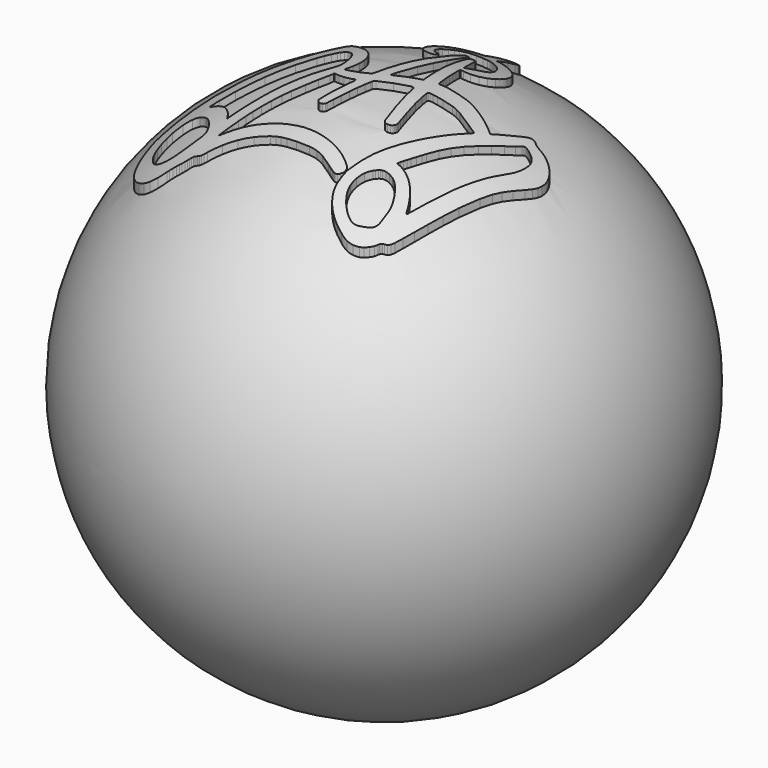
from build123d import *

# Parameters (mm, degrees)
F2_SCALE  = 33.3
F4_DEPTH  = 350
F5_SCALE  = 0.03
F8_SCALE  = 1.4
F9_R      = 2
F10_DEPTH = 25


# Not quite as in the source:
# - ends of sketch curves that miss each other by under 0.0002 mm in the source are joined


with BuildPart() as f1:
    # F0 (on Top) → F1 (revolve)
    with BuildSketch(Plane.XY):
        with BuildLine():
            ThreePointArc((0, 10), (-10, 0), (0, -10))
            Line((0, -10), (0, 10))
        make_face()
    revolve(axis=Axis((0, 0, 0), (0, 1, 0)))


with BuildPart() as f1_1:
    # F2: moved
    add(f1.part.scale(F2_SCALE))

    # F3 (on Top) → F4 (join)
    with BuildSketch(Plane.XY):
        with BuildLine():
            ThreePointArc((16.1837149134, 185.6219143432), (15.1692805921, 185.1870491696), (14.3397748174, 184.4589661515))
            ThreePointArc((14.3397748174, 184.4589661515), (13.6510319308, 183.3784275436), (13.2516433932, 182.1608811178))
            ThreePointArc((13.2516433932, 182.1608811178), (12.7104318622, 179.1680856754), (12.2460595692, 176.1624089195))
            ThreePointArc((12.2460595692, 176.1624089195), (11.7304261477, 172.1284351878), (11.3226162114, 168.0821389815))
            ThreePointArc((11.3226162114, 168.0821389815), (10.8951310079, 162.8117363905), (10.5327134235, 157.536460036))
            Line((10.5327134235, 157.536460036), (9.791164, 145.672526))
            Line((9.791164, 145.672526), (3.780021, 143.498838))
            ThreePointArc((3.780021, 143.498838), (-1.6477610952, 141.1251824988), (-6.7203535297, 138.0651393244))
            ThreePointArc((-6.7203535297, 138.0651393244), (-11.376966369, 134.3574285901), (-15.5191747702, 130.0827038044))
            ThreePointArc((-15.5191747702, 130.0827038044), (-19.0969576158, 125.2903145838), (-22.033620735, 120.0803688722))
            ThreePointArc((-22.033620735, 120.0803688722), (-24.2923210945, 114.5207605988), (-25.8302338375, 108.7202609678))
            ThreePointArc((-25.8302338375, 108.7202609678), (-26.3924557433, 104.1595275807), (-26.2837925551, 99.5655559461))
            ThreePointArc((-26.2837925551, 99.5655559461), (-25.4769738725, 95.4896073492), (-23.8870694152, 91.6507903129))
            ThreePointArc((-23.8870694152, 91.6507903129), (-21.7301657098, 88.5148289409), (-18.934623176, 85.931917761))
            ThreePointArc((-18.934623176, 85.931917761), (-15.6708859709, 84.066137258), (-12.0670000484, 82.9960327237))
            ThreePointArc((-12.0670000484, 82.9960327237), (-9.9514688701, 82.6995503191), (-7.820665005, 82.5477318664))
            ThreePointArc((-7.820665005, 82.5477318664), (-6.2598956775, 82.6218418509), (-4.7338411111, 82.9574763578))
            ThreePointArc((-4.7338411111, 82.9574763578), (-3.6802817431, 83.4443933846), (-2.7901553866, 84.1892094375))
            ThreePointArc((-2.7901553866, 84.1892094375), (-2.1858986044, 85.1009509062), (-1.8924604107, 86.1546550473))
            ThreePointArc((-1.8924604107, 86.1546550473), (-1.8426245804, 86.8806241379), (-1.860013302, 87.6080939788))
            ThreePointArc((-1.860013302, 87.6080939788), (-1.9607246618, 88.1072284011), (-2.1854415077, 88.5641533268))
            ThreePointArc((-2.1854415077, 88.5641533268), (-2.5277112184, 88.9647453673), (-2.9560030801, 89.2716468537))
            ThreePointArc((-2.9560030801, 89.2716468537), (-3.6618204273, 89.6235693148), (-4.392460294, 89.920542189))
            ThreePointArc((-4.392460294, 89.920542189), (-7.1065072138, 91.0410387982), (-9.7123581208, 92.3942217903))
            ThreePointArc((-9.7123581208, 92.3942217903), (-11.4507249242, 93.6626454353), (-12.8778390403, 95.2732859714))
            ThreePointArc((-12.8778390403, 95.2732859714), (-13.8356044552, 97.0406681901), (-14.3428715659, 98.9858249235))
            ThreePointArc((-14.3428715659, 98.9858249235), (-14.521613478, 101.4888433545), (-14.3841001545, 103.9944650183))
            ThreePointArc((-14.3841001545, 103.9944650183), (-13.9482041228, 106.4640083631), (-13.2350706429, 108.8681902312))
            ThreePointArc((-13.2350706429, 108.8681902312), (-12.0847016697, 111.7967649703), (-10.7658611088, 114.6534340541))
            ThreePointArc((-10.7658611088, 114.6534340541), (-9.268237976, 117.4565074493), (-7.6103005428, 120.1678427018))
            ThreePointArc((-7.6103005428, 120.1678427018), (-6.0713916259, 122.2795513115), (-4.3220465667, 124.2205165667))
            ThreePointArc((-4.3220465667, 124.2205165667), (-2.0427283806, 126.2983757659), (0.4185983329, 128.1570475141))
            ThreePointArc((0.4185983329, 128.1570475141), (2.7825294043, 129.5595618954), (5.3085631766, 130.6432455009))
            ThreePointArc((5.3085631766, 130.6432455009), (8.1806159101, 131.4775430213), (11.1293739733, 131.9771082407))
            ThreePointArc((11.1293739733, 131.9771082407), (14.9544272457, 132.2944908395), (18.791164, 132.400393))
            ThreePointArc((18.791164, 132.400393), (21.6806571556, 132.3762113948), (24.5693410001, 132.3036780045))
            ThreePointArc((24.5693410001, 132.3036780045), (26.307751387, 132.1848013044), (28.0336839227, 131.945303557))
            ThreePointArc((28.0336839227, 131.945303557), (29.4825241699, 131.622260103), (30.8949281434, 131.1655213816))
            ThreePointArc((30.8949281434, 131.1655213816), (32.6109340372, 130.4725349399), (34.2911640004, 129.6968200009))
            ThreePointArc((34.2911640004, 129.6968200009), (37.9951081662, 127.5987179258), (41.4287451434, 125.0824961734))
            ThreePointArc((41.4287451434, 125.0824961734), (44.5041115511, 122.2091005808), (47.2099406452, 118.9853187371))
            ThreePointArc((47.2099406452, 118.9853187371), (49.3287125611, 115.6981244902), (51.0020701094, 112.1633380433))
            ThreePointArc((51.0020701094, 112.1633380433), (51.9633429329, 108.8500909146), (52.2845752073, 105.4152019997))
            ThreePointArc((52.2845752073, 105.4152019997), (52.1788202882, 103.3930014318), (51.8679689251, 101.3920390156))
            ThreePointArc((51.8679689251, 101.3920390156), (51.3793933514, 99.7310381661), (50.6292352893, 98.1706238309))
            ThreePointArc((50.6292352893, 98.1706238309), (49.3887670931, 96.267378804), (47.9699187196, 94.4931262474))
            ThreePointArc((47.9699187196, 94.4931262474), (45.1157445833, 91.3136538455), (42.2078228852, 88.1832631085))
            Line((42.2078228852, 88.1832631085), (35.624482, 81.216238))
            Line((35.624482, 81.216238), (31.414756, 95.808316))
            ThreePointArc((31.414756, 95.808316), (30.5747758019, 98.6585264595), (29.7022052286, 101.4989290717))
            ThreePointArc((29.7022052286, 101.4989290717), (28.8907270693, 104.0158337787), (28.0385246844, 106.5192428897))
            ThreePointArc((28.0385246844, 106.5192428897), (27.2982707536, 108.6035005387), (26.5370293603, 110.6801847618))
            ThreePointArc((26.5370293603, 110.6801847618), (26.2437169572, 111.2677894453), (25.8327331947, 111.7800431937))
            ThreePointArc((25.8327331947, 111.7800431937), (25.4802522739, 112.0796118323), (25.0828137789, 112.3163115463))
            ThreePointArc((25.0828137789, 112.3163115463), (24.6227084068, 112.5031852548), (24.141585905, 112.6262294856))
            ThreePointArc((24.141585905, 112.6262294856), (23.6000894231, 112.6925890214), (23.0545419533, 112.6928517741))
            ThreePointArc((23.0545419533, 112.6928517741), (22.4609474828, 112.6292961131), (21.8758000019, 112.5109909925))
            ThreePointArc((21.8758000019, 112.5109909925), (21.2187147252, 112.3098981878), (20.5855640681, 112.0428408591))
            ThreePointArc((20.5855640681, 112.0428408591), (20.1607323375, 111.7679891064), (19.8163702152, 111.3972598449))
            ThreePointArc((19.8163702152, 111.3972598449), (19.5594248386, 110.9371012372), (19.4144355259, 110.4304010782))
            ThreePointArc((19.4144355259, 110.4304010782), (19.3220337791, 109.6802669952), (19.291164, 108.925094))
            ThreePointArc((19.291164, 108.925094), (19.3852916149, 106.0573805668), (19.6672679512, 103.2020119936))
            ThreePointArc((19.6672679512, 103.2020119936), (20.9206581848, 93.8239544773), (22.2043890597, 84.4500020083))
            ThreePointArc((22.2043890597, 84.4500020083), (23.6507956563, 74.229322655), (25.1557427919, 64.0170989687))
            ThreePointArc((25.1557427919, 64.0170989687), (26.6369557977, 54.3850233496), (28.1837279618, 44.7632579937))
            Line((28.1837279618, 44.7632579937), (31.901914, 22.126123))
            Line((31.901914, 22.126123), (26.346539, 19.418249))
            ThreePointArc((26.346539, 19.418249), (24.9715043404, 18.736827914), (23.6055156415, 18.037449689))
            ThreePointArc((23.6055156415, 18.037449689), (21.7119037613, 17.0461943955), (19.8232712195, 16.0454845882))
            ThreePointArc((19.8232712195, 16.0454845882), (17.7770697102, 14.9482118993), (15.7363275839, 13.8408187623))
            ThreePointArc((15.7363275839, 13.8408187623), (13.8353930454, 12.7956894843), (11.9408344366, 11.7390462227))
            ThreePointArc((11.9408344366, 11.7390462227), (10.2357608448, 10.7911533243), (8.5223972402, 9.8583285541))
            ThreePointArc((8.5223972402, 9.8583285541), (7.0602985775, 9.084165839), (5.5872089444, 8.3311271107))
            ThreePointArc((5.5872089444, 8.3311271107), (4.3173161919, 7.6968566116), (3.0447140301, 7.0680399387))
            ThreePointArc((3.0447140301, 7.0680399387), (2.8840367112, 7.0443730497), (2.7395948226, 7.1186288226))
            ThreePointArc((2.7395948226, 7.1186288226), (2.6490578692, 7.2682646369), (2.6382966615, 7.4428270615))
            ThreePointArc((2.6382966615, 7.4428270615), (2.9254660053, 9.0101912635), (3.2173415321, 10.5766859))
            ThreePointArc((3.2173415321, 10.5766859), (3.5670547539, 12.3819405384), (3.9371018372, 14.1831370344))
            ThreePointArc((3.9371018372, 14.1831370344), (4.3905286604, 16.2921707252), (4.8587286662, 18.3979740754))
            ThreePointArc((4.8587286662, 18.3979740754), (7.3036087373, 29.7080586924), (9.5356052963, 41.0620731315))
            ThreePointArc((9.5356052963, 41.0620731315), (11.3297375314, 51.3852863721), (12.8623872203, 61.7505469703))
            ThreePointArc((12.8623872203, 61.7505469703), (14.0102115107, 71.2475265718), (14.8939126099, 80.7727139519))
            ThreePointArc((14.8939126099, 80.7727139519), (15.4313105094, 89.5798061973), (15.6569627413, 98.4003929941))
            ThreePointArc((15.6569627413, 98.4003929941), (15.6890275218, 103.7849560825), (15.7002231557, 109.1696030001))
            ThreePointArc((15.7002231557, 109.1696030001), (15.6481165696, 111.1118828833), (15.4913986894, 113.0485309664))
            ThreePointArc((15.4913986894, 113.0485309664), (15.2950166397, 113.9935034148), (14.919798785, 114.8827448835))
            ThreePointArc((14.919798785, 114.8827448835), (14.4487941297, 115.4056098827), (13.7911639712, 115.6561207748))
            ThreePointArc((13.7911639712, 115.6561207748), (13.3636113076, 115.6929881735), (12.9344749984, 115.694576043))
            ThreePointArc((12.9344749984, 115.694576043), (12.4729567999, 115.6620658314), (12.0145709854, 115.5993090859))
            ThreePointArc((12.0145709854, 115.5993090859), (11.5887291287, 115.5117299525), (11.1697992405, 115.3955012347))
            ThreePointArc((11.1697992405, 115.3955012347), (10.8507606005, 115.2707067502), (10.5516966736, 115.1036135006))
            ThreePointArc((10.5516966736, 115.1036135006), (10.1768291835, 114.7430744846), (9.9606132353, 114.2700369423))
            ThreePointArc((9.9606132353, 114.2700369423), (9.2991267255, 111.5350836806), (8.6559357265, 108.7957700633))
            ThreePointArc((8.6559357265, 108.7957700633), (7.9317638824, 105.5484568402), (7.2587524522, 102.2901561087))
            ThreePointArc((7.2587524522, 102.2901561087), (6.5246468823, 98.4896960964), (5.8286649433, 94.6820700101))
            ThreePointArc((5.8286649433, 94.6820700101), (3.2390112568, 80.4502627726), (0.5295064699, 66.2407861034))
            ThreePointArc((0.5295064699, 66.2407861034), (-2.6948106938, 49.9526915591), (-6.0100623355, 33.6828620693))
            ThreePointArc((-6.0100623355, 33.6828620693), (-9.4598472935, 17.0258658736), (-12.9233232351, 0.371711049))
            ThreePointArc((-12.9233232351, 0.371711049), (-13.3605462648, -0.8244338456), (-14.1215245934, -1.8456284066))
            ThreePointArc((-14.1215245934, -1.8456284066), (-14.298805794, -1.991284186), (-14.5009786768, -2.0997757755))
            ThreePointArc((-14.5009786768, -2.0997757755), (-15.4717200684, -2.5016106982), (-16.4443961129, -2.8987397215))
            ThreePointArc((-16.4443961129, -2.8987397215), (-17.5933724189, -3.357741385), (-18.7470091084, -3.804900716))
            ThreePointArc((-18.7470091084, -3.804900716), (-20.067808676, -4.3038158125), (-21.3920379976, -4.7935550064))
            ThreePointArc((-21.3920379976, -4.7935550064), (-24.693503143, -5.8648357681), (-28.0651240346, -6.6891458318))
            ThreePointArc((-28.0651240346, -6.6891458318), (-31.925581958, -7.3800215193), (-35.8164370636, -7.8716423663))
            ThreePointArc((-35.8164370636, -7.8716423663), (-39.1746262166, -8.1377523396), (-42.5410049916, -8.2632235157))
            ThreePointArc((-42.5410049916, -8.2632235157), (-43.3114521438, -7.86442986), (-43.4025439079, -7.0016860377))
            ThreePointArc((-43.4025439079, -7.0016860377), (-41.8130495855, -2.5451973195), (-40.641365393, 2.0388990813))
            ThreePointArc((-40.641365393, 2.0388990813), (-39.9495299937, 6.5434580932), (-39.7259944757, 11.0953499988))
            ThreePointArc((-39.7259944757, 11.0953499988), (-39.9736025735, 15.4953280542), (-40.6907613549, 19.8435231423))
            ThreePointArc((-40.6907613549, 19.8435231423), (-41.858302321, 23.9893435365), (-43.493257789, 27.974051622))
            ThreePointArc((-43.493257789, 27.974051622), (-45.8358535005, 32.1828815852), (-48.6740508408, 36.0747501317))
            ThreePointArc((-48.6740508408, 36.0747501317), (-52.0247211521, 39.6828979629), (-55.7654615455, 42.8848635969))
            ThreePointArc((-55.7654615455, 42.8848635969), (-59.9662832556, 45.7305331977), (-64.4556810239, 48.0948609477))
            ThreePointArc((-64.4556810239, 48.0948609477), (-69.3196757609, 50.0321037845), (-74.3538649509, 51.4702602117))
            ThreePointArc((-74.3538649509, 51.4702602117), (-77.5971585248, 52.060235073), (-80.8820409982, 52.3369490499))
            ThreePointArc((-80.8820409982, 52.3369490499), (-82.9473411991, 52.0505112999), (-84.7913459515, 51.0772909374))
            ThreePointArc((-84.7913459515, 51.0772909374), (-86.7701676601, 49.231226631), (-88.3813987235, 47.0569168318))
            ThreePointArc((-88.3813987235, 47.0569168318), (-91.9069280027, 41.156453721), (-95.3378537719, 35.2004844365))
            ThreePointArc((-95.3378537719, 35.2004844365), (-99.490595888, 28.010177071), (-103.7735608571, 20.8966689122))
            ThreePointArc((-103.7735608571, 20.8966689122), (-108.7531882179, 12.9064292235), (-113.8324117533, 4.9791278397))
            ThreePointArc((-113.8324117533, 4.9791278397), (-120.3277806536, -4.917768916), (-126.9160680745, -14.7530549496))
            ThreePointArc((-126.9160680745, -14.7530549496), (-135.9712787588, -28.0792936439), (-145.0774889955, -41.3707350031))
            ThreePointArc((-145.0774889955, -41.3707350031), (-153.20486316, -53.2582674065), (-161.2634160329, -65.1925609779))
            ThreePointArc((-161.2634160329, -65.1925609779), (-167.2375766356, -74.2246819748), (-173.0909778416, -83.3355271003))
            ThreePointArc((-173.0909778416, -83.3355271003), (-177.563070075, -90.5376655525), (-181.9087261093, -97.816791936))
            ThreePointArc((-181.9087261093, -97.816791936), (-185.2879018817, -103.8114638517), (-188.4712984623, -109.9123577682))
            ThreePointArc((-188.4712984623, -109.9123577682), (-190.2540089518, -113.5255935339), (-191.9903037715, -117.1613616376))
            ThreePointArc((-191.9903037715, -117.1613616376), (-192.7930450128, -119.0638070124), (-193.4417981706, -121.024115951))
            ThreePointArc((-193.4417981706, -121.024115951), (-193.879582697, -122.8798340455), (-194.1371780105, -124.7690109991))
            ThreePointArc((-194.1371780105, -124.7690109991), (-194.3739822626, -127.8947928847), (-194.5368125893, -131.0253000165))
            ThreePointArc((-194.5368125893, -131.0253000165), (-194.3823750031, -138.2436150808), (-193.3429853893, -145.3883748724))
            ThreePointArc((-193.3429853893, -145.3883748724), (-191.4753146978, -151.7792971079), (-188.633494165, -157.8006040943))
            ThreePointArc((-188.633494165, -157.8006040943), (-184.9737479765, -163.1446659147), (-180.4982857453, -167.8268637135))
            ThreePointArc((-180.4982857453, -167.8268637135), (-175.1554159196, -171.9267200048), (-169.2776890554, -175.2141821185))
            ThreePointArc((-169.2776890554, -175.2141821185), (-165.0035576963, -176.9300756149), (-160.5646198449, -178.1582122865))
            ThreePointArc((-160.5646198449, -178.1582122865), (-156.3827311483, -178.7545456112), (-152.1585579711, -178.741581383))
            ThreePointArc((-152.1585579711, -178.741581383), (-147.9897477257, -178.1200783399), (-143.9546518648, -176.9021923531))
            ThreePointArc((-143.9546518648, -176.9021923531), (-139.7773284426, -175.0248897158), (-135.8390842742, -172.6872565926))
            ThreePointArc((-135.8390842742, -172.6872565926), (-134.6684659752, -171.9217841853), (-133.4780123266, -171.1875394545))
            ThreePointArc((-133.4780123266, -171.1875394545), (-132.02357575, -170.3317183771), (-130.556336222, -169.4980376022))
            ThreePointArc((-130.556336222, -169.4980376022), (-129.066933111, -168.681346713), (-127.565344933, -167.8872821291))
            ThreePointArc((-127.565344933, -167.8872821291), (-126.2831509664, -167.2417808419), (-124.9852508797, -166.628471263))
            ThreePointArc((-124.9852508797, -166.628471263), (-123.7657782561, -166.0449605457), (-122.5672611004, -165.4195368155))
            ThreePointArc((-122.5672611004, -165.4195368155), (-121.3125176022, -164.7133256706), (-120.0785574692, -163.9713972443))
            ThreePointArc((-120.0785574692, -163.9713972443), (-118.9647815028, -163.2570511422), (-117.8723278692, -162.5105041855))
            ThreePointArc((-117.8723278692, -162.5105041855), (-117.1100421405, -161.9293776695), (-116.3931727882, -161.2930712214))
            ThreePointArc((-116.3931727882, -161.2930712214), (-115.596607323, -160.5872014341), (-114.748597957, -159.9440460614))
            ThreePointArc((-114.748597957, -159.9440460614), (-113.9964520554, -159.4894929311), (-113.190213915, -159.1397472385))
            ThreePointArc((-113.190213915, -159.1397472385), (-112.2874291011, -158.8783332711), (-111.3597539314, -158.7274146769))
            ThreePointArc((-111.3597539314, -158.7274146769), (-110.0967660617, -158.631579334), (-108.830551, -158.599607))
            ThreePointArc((-108.830551, -158.599607), (-107.4591786164, -158.5559107374), (-106.0933700077, -158.4249969397))
            ThreePointArc((-106.0933700077, -158.4249969397), (-105.0528819949, -158.2192738025), (-104.0497489931, -157.8748010163))
            ThreePointArc((-104.0497489931, -157.8748010163), (-102.9942635093, -157.3584629036), (-102.0036018033, -156.7266052731))
            ThreePointArc((-102.0036018033, -156.7266052731), (-100.5566526639, -155.6476823357), (-99.146214049, -154.5214499407))
            ThreePointArc((-99.146214049, -154.5214499407), (-93.1943058803, -149.9369406786), (-86.9443147957, -145.7679423301))
            ThreePointArc((-86.9443147957, -145.7679423301), (-80.2377344142, -141.9002504552), (-73.3036320885, -138.4570708068))
            ThreePointArc((-73.3036320885, -138.4570708068), (-65.757943521, -135.2619707968), (-58.0384350021, -132.5132859934))
            ThreePointArc((-58.0384350021, -132.5132859934), (-49.5569866342, -129.9858687202), (-40.9673479529, -127.8549272106))
            ThreePointArc((-40.9673479529, -127.8549272106), (-37.922317166, -127.2275267291), (-34.8579750625, -126.7025015945))
            ThreePointArc((-34.8579750625, -126.7025015945), (-31.998971604, -126.3230465362), (-29.1265679853, -126.0638472123))
            ThreePointArc((-29.1265679853, -126.0638472123), (-25.4717422355, -125.8628877022), (-21.8127060078, -125.7649593825))
            ThreePointArc((-21.8127060078, -125.7649593825), (-15.7608917275, -125.7089235101), (-9.7088359997, -125.694173658))
            ThreePointArc((-9.7088359997, -125.694173658), (-1.4052780416, -125.7897254934), (6.8944249967, -126.0601590774))
            ThreePointArc((6.8944249967, -126.0601590774), (12.1704491822, -126.4887139133), (17.3987960722, -127.3160466341))
            ThreePointArc((17.3987960722, -127.3160466341), (22.0222060987, -128.4519660894), (26.5216057179, -130.0081267082))
            ThreePointArc((26.5216057179, -130.0081267082), (32.2284552595, -132.4226478092), (37.8276242244, -135.0773325516))
            ThreePointArc((37.8276242244, -135.0773325516), (39.8180636809, -136.0543732185), (41.8232317536, -137.0008185326))
            ThreePointArc((41.8232317536, -137.0008185326), (43.666667609, -137.8312508638), (45.5264859584, -138.6243141003))
            ThreePointArc((45.5264859584, -138.6243141003), (47.085200235, -139.2562693288), (48.653583967, -139.8638300871))
            ThreePointArc((48.653583967, -139.8638300871), (49.2874829785, -140.0401776207), (49.942765, -140.099607))
            ThreePointArc((49.942765, -140.099607), (51.3009933898, -139.9453099932), (52.5900021043, -139.4902842146))
            ThreePointArc((52.5900021043, -139.4902842146), (53.8726217093, -138.7226734394), (55.0033189099, -137.7449909125))
            ThreePointArc((55.0033189099, -137.7449909125), (55.9584400613, -136.5762073319), (56.6997423526, -135.261375705))
            ThreePointArc((56.6997423526, -135.261375705), (57.1416068628, -133.9307841967), (57.291164, -132.536743))
            ThreePointArc((57.291164, -132.536743), (57.237707326, -131.5541979548), (57.0779690168, -130.5832519963))
            ThreePointArc((57.0779690168, -130.5832519963), (56.8277685223, -129.8099854498), (56.4352883269, -129.0982967766))
            ThreePointArc((56.4352883269, -129.0982967766), (55.8234411064, -128.3202541625), (55.1132866195, -127.6307704484))
            ThreePointArc((55.1132866195, -127.6307704484), (53.8436472357, -126.5878348415), (52.5411638957, -125.5862181403))
            ThreePointArc((52.5411638957, -125.5862181403), (47.475600047, -122.1621367631), (42.1222817805, -119.208113444))
            ThreePointArc((42.1222817805, -119.208113444), (35.9652987585, -116.4160361686), (29.635663052, -114.041199846))
            ThreePointArc((29.635663052, -114.041199846), (22.6188796119, -111.9113493104), (15.484156052, -110.2180587463))
            ThreePointArc((15.484156052, -110.2180587463), (7.8051826054, -108.848087575), (0.0660969851, -107.8734041489))
            ThreePointArc((0.0660969851, -107.8734041489), (-11.5578912242, -107.2430315126), (-23.1910900201, -107.6710007556))
            ThreePointArc((-23.1910900201, -107.6710007556), (-35.7976050733, -109.1572942696), (-48.2687728762, -111.5244155466))
            ThreePointArc((-48.2687728762, -111.5244155466), (-60.5764222456, -114.7685170173), (-72.6267360643, -118.8663658307))
            ThreePointArc((-72.6267360643, -118.8663658307), (-83.4075588982, -123.5189390406), (-93.7312352296, -129.113068618))
            ThreePointArc((-93.7312352296, -129.113068618), (-95.2577593466, -130.022900739), (-96.7909421062, -130.9214668173))
            ThreePointArc((-96.7909421062, -130.9214668173), (-98.0735574173, -131.6559717717), (-99.3654159561, -132.3740950803))
            ThreePointArc((-99.3654159561, -132.3740950803), (-100.4639476171, -132.9729309302), (-101.5647409619, -133.5675990709))
            ThreePointArc((-101.5647409619, -133.5675990709), (-101.6612175085, -133.5654141524), (-101.708836, -133.48148))
            ThreePointArc((-101.708836, -133.48148), (-101.6910575573, -133.3212945765), (-101.6385871349, -133.1689059361))
            ThreePointArc((-101.6385871349, -133.1689059361), (-101.0782228381, -131.9878147807), (-100.5158437749, -130.8076816299))
            ThreePointArc((-100.5158437749, -130.8076816299), (-99.8642513231, -129.4541470073), (-99.2042778166, -128.1046790904))
            ThreePointArc((-99.2042778166, -128.1046790904), (-98.4290257596, -126.5396873074), (-97.6475821287, -124.9777779353))
            ThreePointArc((-97.6475821287, -124.9777779353), (-96.5946988144, -122.8560100638), (-95.5641559418, -120.7233020277))
            ThreePointArc((-95.5641559418, -120.7233020277), (-94.0022911598, -117.4342232392), (-92.4505441515, -114.1403589289))
            ThreePointArc((-92.4505441515, -114.1403589289), (-90.7153599133, -110.4275005562), (-88.9916419708, -106.7093050135))
            ThreePointArc((-88.9916419708, -106.7093050135), (-87.3190830878, -103.0710186046), (-85.6585760176, -99.427215992))
            ThreePointArc((-85.6585760176, -99.427215992), (-83.7859611792, -95.3699389506), (-81.8609478505, -91.3372590725))
            ThreePointArc((-81.8609478505, -91.3372590725), (-79.4143308998, -86.3392952904), (-76.9339135573, -81.3580197201))
            ThreePointArc((-76.9339135573, -81.3580197201), (-74.3549780316, -76.2653944696), (-71.7417980187, -71.1902559903))
            ThreePointArc((-71.7417980187, -71.1902559903), (-69.4384958804, -66.8090452768), (-67.0901819752, -62.4517950135))
            ThreePointArc((-67.0901819752, -62.4517950135), (-63.5541885564, -55.8402761879), (-60.1291065795, -49.1706252115))
            ThreePointArc((-60.1291065795, -49.1706252115), (-56.8951651545, -42.59575666), (-53.7793826385, -35.9640771659))
            ThreePointArc((-53.7793826385, -35.9640771659), (-51.1372353945, -30.1211161127), (-48.5607036818, -24.2489257054))
            ThreePointArc((-48.5607036818, -24.2489257054), (-47.93781126, -22.2881655457), (-47.7180140094, -20.242618))
            ThreePointArc((-47.7180140094, -20.242618), (-47.6866978572, -19.9784340952), (-47.5978704944, -19.7276682453))
            ThreePointArc((-47.5978704944, -19.7276682453), (-47.4643858192, -19.5431886932), (-47.275807769, -19.4155595169))
            ThreePointArc((-47.275807769, -19.4155595169), (-47.022785308, -19.3418905312), (-46.7592679429, -19.3394075545))
            ThreePointArc((-46.7592679429, -19.3394075545), (-46.4145564122, -19.4047193248), (-46.0800829849, -19.5106399606))
            ThreePointArc((-46.0800829849, -19.5106399606), (-43.1858515948, -20.4596333373), (-40.2119128983, -21.1175484007))
            ThreePointArc((-40.2119128983, -21.1175484007), (-36.723738698, -21.5947008978), (-33.2120829862, -21.846311648))
            ThreePointArc((-33.2120829862, -21.846311648), (-29.6737492069, -21.8717876005), (-26.1410780089, -21.6700719003))
            ThreePointArc((-26.1410780089, -21.6700719003), (-23.0697693824, -21.247363637), (-20.0525718819, -20.5345254112))
            ThreePointArc((-20.0525718819, -20.5345254112), (-19.4468474642, -20.6109105717), (-19.084589067, -21.1023430157))
            ThreePointArc((-19.084589067, -21.1023430157), (-18.9430855771, -22.1618326663), (-19.0093187401, -23.2286760418))
            ThreePointArc((-19.0093187401, -23.2286760418), (-19.4681665954, -25.7552544106), (-20.0289718034, -28.261174803))
            ThreePointArc((-20.0289718034, -28.261174803), (-21.8192933551, -35.5226759663), (-23.6285763044, -42.7794759237))
            ThreePointArc((-23.6285763044, -42.7794759237), (-24.7249244466, -47.2109922121), (-25.7936169536, -51.649259011))
            ThreePointArc((-25.7936169536, -51.649259011), (-26.6889739902, -55.5011427518), (-27.5474355142, -59.3614168882))
            ThreePointArc((-27.5474355142, -59.3614168882), (-28.2627324882, -62.6803264695), (-28.9663104022, -66.0017401255))
            ThreePointArc((-28.9663104022, -66.0017401255), (-29.0129846825, -66.5645713801), (-28.919805713, -67.1215949144))
            ThreePointArc((-28.919805713, -67.1215949144), (-28.2842355826, -68.4500491849), (-27.2710210934, -69.5187571214))
            ThreePointArc((-27.2710210934, -69.5187571214), (-25.8566439297, -70.3750412424), (-24.2880199884, -70.8976349455))
            ThreePointArc((-24.2880199884, -70.8976349455), (-22.6370376768, -71.0621254424), (-20.9903070315, -70.8594488674))
            ThreePointArc((-20.9903070315, -70.8594488674), (-19.6163073104, -70.2993253837), (-18.4762862242, -69.3496068023))
            ThreePointArc((-18.4762862242, -69.3496068023), (-17.9945458178, -68.6712789333), (-17.664695396, -67.9074718763))
            ThreePointArc((-17.664695396, -67.9074718763), (-16.5384590313, -64.2681667173), (-15.4311923539, -60.6230451944))
            ThreePointArc((-15.4311923539, -60.6230451944), (-14.1613597181, -56.3173468657), (-12.9391033599, -51.9979021773))
            ThreePointArc((-12.9391033599, -51.9979021773), (-11.5892211853, -47.0537010718), (-10.2761107689, -42.0996070603))
            ThreePointArc((-10.2761107689, -42.0996070603), (-8.9814934643, -37.1459429181), (-7.6844483946, -32.1929138966))
            ThreePointArc((-7.6844483946, -32.1929138966), (-6.5490429829, -27.8679228913), (-5.4104643641, -23.5437661677))
            ThreePointArc((-5.4104643641, -23.5437661677), (-4.431724195, -19.8343904293), (-3.4518924379, -16.1253028843))
            ThreePointArc((-3.4518924379, -16.1253028843), (-3.2622195861, -15.4307074626), (-3.0612499127, -14.7392960262))
            ThreePointArc((-3.0612499127, -14.7392960262), (-2.129536934, -13.0381334806), (-0.5850247262, -11.8648795822))
            ThreePointArc((-0.5850247262, -11.8648795822), (7.4707042881, -8.1283305445), (15.5654921953, -4.4771694391))
            ThreePointArc((15.5654921953, -4.4771694391), (23.7398033717, -0.889987303), (31.9489529534, 2.6167351105))
            ThreePointArc((31.9489529534, 2.6167351105), (33.6918666155, 2.899267892), (35.3703910352, 2.3514280569))
            ThreePointArc((35.3703910352, 2.3514280569), (35.5566586924, 2.1848581186), (35.6740518319, 1.9642679456))
            ThreePointArc((35.6740518319, 1.9642679456), (35.8762294486, 1.3103440022), (36.061139733, 0.6513291953))
            ThreePointArc((36.061139733, 0.6513291953), (36.26314999, -0.1621047432), (36.4374231899, -0.981928963))
            ThreePointArc((36.4374231899, -0.981928963), (36.6063276397, -1.9077239631), (36.7529385065, -2.8373100718))
            ThreePointArc((36.7529385065, -2.8373100718), (37.6446472321, -8.373665741), (38.7051243622, -13.880186133))
            ThreePointArc((38.7051243622, -13.880186133), (40.9607034561, -24.5673034397), (43.2689418368, -35.2431710357))
            ThreePointArc((43.2689418368, -35.2431710357), (45.8461272941, -46.9921813164), (48.4358832749, -58.7384271603))
            ThreePointArc((48.4358832749, -58.7384271603), (48.8104411302, -59.8097538209), (49.4266262823, -60.7628277657))
            ThreePointArc((49.4266262823, -60.7628277657), (50.2525608671, -61.4796427144), (51.2647969457, -61.8936112373))
            ThreePointArc((51.2647969457, -61.8936112373), (52.6410377476, -62.0925439858), (54.0313259655, -62.0658696583))
            ThreePointArc((54.0313259655, -62.0658696583), (55.503671983, -61.8034613245), (56.9194837467, -61.3216544072))
            ThreePointArc((56.9194837467, -61.3216544072), (58.0977285914, -60.6671875239), (59.1168501049, -59.7851560986))
            ThreePointArc((59.1168501049, -59.7851560986), (59.55008435, -59.2915367781), (59.9489374034, -58.7697435752))
            ThreePointArc((59.9489374034, -58.7697435752), (60.3189454936, -58.213140171), (60.652459214, -57.6339321142))
            ThreePointArc((60.652459214, -57.6339321142), (60.915070309, -57.0992856211), (61.1410199596, -56.548142985))
            ThreePointArc((61.1410199596, -56.548142985), (61.2533302438, -56.1367176315), (61.291164, -55.71192))
            ThreePointArc((61.291164, -55.71192), (61.2635825051, -55.0887422425), (61.1810530137, -54.4704379975))
            ThreePointArc((61.1810530137, -54.4704379975), (60.739257562, -52.0200600057), (60.2903282561, -49.5709789527))
            ThreePointArc((60.2903282561, -49.5709789527), (59.7478982488, -46.6807821036), (59.1894587401, -43.7936358547))
            ThreePointArc((59.1894587401, -43.7936358547), (58.5430275787, -40.5337483179), (57.8840642292, -37.2763709532))
            ThreePointArc((57.8840642292, -37.2763709532), (55.9130545378, -27.4898736257), (53.996625103, -17.6925419801))
            ThreePointArc((53.996625103, -17.6925419801), (52.8274566906, -11.2993254233), (51.7800238499, -4.885040023))
            ThreePointArc((51.7800238499, -4.885040023), (51.1154910958, -0.348355952), (50.5137886788, 4.1970879597))
            ThreePointArc((50.5137886788, 4.1970879597), (50.6261754498, 5.2861516335), (51.2057709817, 6.2150000183))
            ThreePointArc((51.2057709817, 6.2150000183), (51.7316784384, 6.5882253271), (52.3513080566, 6.7669284996))
            ThreePointArc((52.3513080566, 6.7669284996), (54.2004946993, 6.9550049108), (56.0534360253, 7.1015396271))
            ThreePointArc((56.0534360253, 7.1015396271), (58.6398980813, 7.2448599344), (61.2291099892, 7.3242855898))
            ThreePointArc((61.2291099892, 7.3242855898), (64.9064262575, 7.3752249203), (68.5840509998, 7.3932804491))
            ThreePointArc((68.5840509998, 7.3932804491), (74.4014010958, 7.3540957103), (80.2175899968, 7.2314408857))
            ThreePointArc((80.2175899968, 7.2314408857), (83.0482951328, 7.0090568789), (85.8425150109, 6.5043970467))
            ThreePointArc((85.8425150109, 6.5043970467), (88.826522043, 5.6879843925), (91.7394332619, 4.6459786524))
            ThreePointArc((91.7394332619, 4.6459786524), (99.2748115979, 1.5936546442), (106.7911642673, -1.5052243574))
            ThreePointArc((106.7911642673, -1.5052243574), (108.9271172862, -2.3925802095), (111.0637817722, -3.2782215502))
            ThreePointArc((111.0637817722, -3.2782215502), (112.9273228851, -4.0484610291), (114.7917929302, -4.8164491697))
            ThreePointArc((114.7917929302, -4.8164491697), (116.3949092477, -5.4752156884), (117.9983321531, -6.1332356266))
            ThreePointArc((117.9983321531, -6.1332356266), (118.287886316, -6.2472407023), (118.5805411484, -6.3530325706))
            ThreePointArc((118.5805411484, -6.3530325706), (118.7443621044, -6.5063609495), (118.7397318253, -6.7306939177))
            ThreePointArc((118.7397318253, -6.7306939177), (118.0821669931, -8.10842605), (117.410544653, -9.4793603241))
            ThreePointArc((117.410544653, -9.4793603241), (116.567582792, -11.1310347744), (115.6876550529, -12.7633154756))
            ThreePointArc((115.6876550529, -12.7633154756), (114.6011264155, -14.6953093854), (113.4890868701, -16.6127329235))
            ThreePointArc((113.4890868701, -16.6127329235), (112.0308941285, -19.1074919978), (110.5888878646, -21.6116419226))
            ThreePointArc((110.5888878646, -21.6116419226), (108.581802608, -25.1332502247), (106.5832592405, -28.6597131359))
            ThreePointArc((106.5832592405, -28.6597131359), (104.4152533351, -32.5068028916), (102.2564953098, -36.3590896143))
            ThreePointArc((102.2564953098, -36.3590896143), (100.2420143008, -39.9764230324), (98.2380748975, -43.5996069435))
            ThreePointArc((98.2380748975, -43.5996069435), (96.1615087685, -47.3647499895), (94.0829917357, -51.1288164065))
            ThreePointArc((94.0829917357, -51.1288164065), (91.7087632499, -55.424), (89.3330404598, -59.7183572545))
            ThreePointArc((89.3330404598, -59.7183572545), (87.0335714153, -63.8714433591), (84.7326410432, -68.0237200239))
            ThreePointArc((84.7326410432, -68.0237200239), (82.9080616199, -71.3123010274), (81.0811866273, -74.5996073489))
            ThreePointArc((81.0811866273, -74.5996073489), (77.1756304529, -81.8252266527), (73.4453793066, -89.1428881517))
            ThreePointArc((73.4453793066, -89.1428881517), (70.463489184, -95.4770677052), (67.7293749935, -101.9220749974))
            ThreePointArc((67.7293749935, -101.9220749974), (65.3354048943, -108.2526296552), (63.2001678068, -114.6750729401))
            ThreePointArc((63.2001678068, -114.6750729401), (61.0907047094, -121.8572998694), (59.1977685343, -129.0996068857))
            ThreePointArc((59.1977685343, -129.0996068857), (58.7155219026, -131.5492575633), (58.4616752936, -134.0329870163))
            ThreePointArc((58.4616752936, -134.0329870163), (58.3501032707, -137.2841010216), (58.376969432, -140.5370179872))
            ThreePointArc((58.376969432, -140.5370179872), (58.5437512694, -143.8138085619), (58.8500216398, -147.0805150415))
            ThreePointArc((58.8500216398, -147.0805150415), (59.2567424644, -149.6461584638), (59.8794210294, -152.1681059914))
            ThreePointArc((59.8794210294, -152.1681059914), (61.4126484575, -156.4333894478), (63.4503064018, -160.482016348))
            ThreePointArc((63.4503064018, -160.482016348), (66.0558445179, -164.4656139977), (69.0634288442, -168.1551011412))
            ThreePointArc((69.0634288442, -168.1551011412), (72.6014971104, -171.6895607473), (76.4724249591, -174.8559860554))
            ThreePointArc((76.4724249591, -174.8559860554), (80.7986134694, -177.7662638509), (85.3628880374, -180.2867839247))
            ThreePointArc((85.3628880374, -180.2867839247), (89.8664357822, -182.3566666418), (94.4857180178, -184.1534939498))
            ThreePointArc((94.4857180178, -184.1534939498), (98.1892590099, -185.2116669326), (101.9961230179, -185.7979538021))
            ThreePointArc((101.9961230179, -185.7979538021), (105.3951179449, -185.8486280906), (108.7633799035, -185.3897755485))
            ThreePointArc((108.7633799035, -185.3897755485), (112.2292645089, -184.4160568758), (115.5443630561, -183.0122741122))
            ThreePointArc((115.5443630561, -183.0122741122), (117.4952977899, -181.9332903233), (119.3505719274, -180.6970419002))
            ThreePointArc((119.3505719274, -180.6970419002), (121.3776378174, -179.1352849185), (123.3161484472, -177.4648784911))
            ThreePointArc((123.3161484472, -177.4648784911), (125.0857526406, -175.7616607129), (126.7585197901, -173.9632448153))
            ThreePointArc((126.7585197901, -173.9632448153), (127.9207430816, -172.4719200938), (128.8974915637, -170.8530392958))
            ThreePointArc((128.8974915637, -170.8530392958), (129.2570475309, -170.2546347434), (129.6831548953, -169.7016419092))
            ThreePointArc((129.6831548953, -169.7016419092), (130.2531984589, -169.0870900158), (130.8632040698, -168.5121840792))
            ThreePointArc((130.8632040698, -168.5121840792), (131.5263611974, -167.9659245187), (132.2242608765, -167.4648128153))
            ThreePointArc((132.2242608765, -167.4648128153), (132.8775368088, -167.0712019821), (133.5650698173, -166.7410545683))
            ThreePointArc((133.5650698173, -166.7410545683), (135.1171314216, -165.9664319053), (136.5604258717, -165.0042278314))
            ThreePointArc((136.5604258717, -165.0042278314), (137.7706074555, -163.9272550787), (138.8020785717, -162.6780644026))
            ThreePointArc((138.8020785717, -162.6780644026), (140.0144805187, -160.7904241937), (141.061788858, -158.8064259326))
            ThreePointArc((141.061788858, -158.8064259326), (142.8494724934, -154.9660623079), (144.580001611, -151.0996072681))
            ThreePointArc((144.580001611, -151.0996072681), (147.1171744125, -145.0819041286), (149.4798028822, -138.9935559562))
            ThreePointArc((149.4798028822, -138.9935559562), (152.1370487514, -131.6518442683), (154.6693622853, -124.2661097617))
            ThreePointArc((154.6693622853, -124.2661097617), (157.4060203193, -115.8452729244), (160.0143212149, -107.3837980645))
            ThreePointArc((160.0143212149, -107.3837980645), (162.7575087274, -98.0442712795), (165.3935455463, -88.6739378752))
            ThreePointArc((165.3935455463, -88.6739378752), (168.826434421, -76.2801253409), (172.3016404764, -63.8981118521))
            ThreePointArc((172.3016404764, -63.8981118521), (174.3630687453, -56.8202540268), (176.538569949, -49.7766219838))
            ThreePointArc((176.538569949, -49.7766219838), (178.3228475955, -44.3988594789), (180.2433148701, -39.0682139513))
            ThreePointArc((180.2433148701, -39.0682139513), (182.4436097648, -33.3730379486), (184.7592665156, -27.7237847957))
            ThreePointArc((184.7592665156, -27.7237847957), (187.3550570533, -21.4578253559), (189.8699420965, -15.1589580378))
            ThreePointArc((189.8699420965, -15.1589580378), (191.3797694483, -11.0372517517), (192.7043340922, -6.8523300269))
            ThreePointArc((192.7043340922, -6.8523300269), (193.530924968, -3.6261533571), (194.1402225784, -0.351977936))
            ThreePointArc((194.1402225784, -0.351977936), (194.4863702249, 2.7653629148), (194.5823845492, 5.9003930051))
            ThreePointArc((194.5823845492, 5.9003930051), (193.9467970003, 12.0958183393), (192.1781030023, 18.0673330009))
            ThreePointArc((192.1781030023, 18.0673330009), (189.2978434253, 23.7928234234), (185.4876400925, 28.9464130814))
            ThreePointArc((185.4876400925, 28.9464130814), (180.8876452841, 33.3439190163), (175.6029469737, 36.8893349525))
            ThreePointArc((175.6029469737, 36.8893349525), (169.9893790557, 39.3169372756), (164.0137349883, 40.6196559015))
            ThreePointArc((164.0137349883, 40.6196559015), (162.9505868535, 40.7745681528), (161.897267121, 40.9862265285))
            ThreePointArc((161.897267121, 40.9862265285), (160.8828883324, 41.249551381), (159.8854019231, 41.570993783))
            ThreePointArc((159.8854019231, 41.570993783), (159.0316962121, 41.9036867853), (158.2002242815, 42.2885925617))
            ThreePointArc((158.2002242815, 42.2885925617), (157.6357489497, 42.6306028389), (157.1331600375, 43.0583970375))
            ThreePointArc((157.1331600375, 43.0583970375), (156.236385366, 43.7989323515), (155.2157391971, 44.35649746))
            ThreePointArc((155.2157391971, 44.35649746), (154.1193160808, 44.7034681785), (152.9762220004, 44.8294370385))
            ThreePointArc((152.9762220004, 44.8294370385), (151.8665621257, 44.7281044614), (150.8007388291, 44.4030904061))
            ThreePointArc((150.8007388291, 44.4030904061), (149.8588544962, 43.8751237541), (149.0584421231, 43.1503928915))
            ThreePointArc((149.0584421231, 43.1503928915), (148.641491834, 42.6355895366), (148.2689420919, 42.0877969429))
            ThreePointArc((148.2689420919, 42.0877969429), (147.6368041366, 41.0513177162), (147.0209505168, 40.0050807012))
            ThreePointArc((147.0209505168, 40.0050807012), (146.3187726055, 38.7669112896), (145.6372968247, 37.5172280937))
            ThreePointArc((145.6372968247, 37.5172280937), (144.9531230011, 36.2138843914), (144.288638533, 34.9003932319))
            ThreePointArc((144.288638533, 34.9003932319), (143.4652014739, 33.2794742987), (142.6120618468, 31.6739900832))
            ThreePointArc((142.6120618468, 31.6739900832), (141.376019346, 29.4168637686), (140.1248284449, 27.1680993113))
            ThreePointArc((140.1248284449, 27.1680993113), (138.7398628705, 24.7176466791), (137.3385979295, 22.2764780408))
            ThreePointArc((137.3385979295, 22.2764780408), (136.0012155124, 19.9855560165), (134.6456447532, 17.705349148))
            Line((134.6456447532, 17.705349148), (128.229754, 7.010305))
            Line((128.229754, 7.010305), (121.8221, 11.489575))
            ThreePointArc((121.8221, 11.489575), (118.292516701, 13.8191390884), (114.6435921446, 15.9569362626))
            ThreePointArc((114.6435921446, 15.9569362626), (110.2210787273, 18.2991977167), (105.7250388684, 20.4970237195))
            ThreePointArc((105.7250388684, 20.4970237195), (101.1764238702, 22.5407121339), (96.5639481057, 24.4358712695))
            ThreePointArc((96.5639481057, 24.4358712695), (92.6406330214, 25.8505956206), (88.645348113, 27.0470674191))
            ThreePointArc((88.645348113, 27.0470674191), (84.7519198615, 27.9277560629), (80.7994809645, 28.4868826448))
            ThreePointArc((80.7994809645, 28.4868826448), (75.1603929861, 28.9654811468), (69.5095479944, 29.27583686))
            ThreePointArc((69.5095479944, 29.27583686), (63.8795483536, 29.4176489364), (58.2478170029, 29.3929788496))
            ThreePointArc((58.2478170029, 29.3929788496), (54.3961014382, 29.1496129169), (50.5806051113, 28.569158436))
            ThreePointArc((50.5806051113, 28.569158436), (49.3070954349, 28.3335524543), (48.0283099591, 28.1285042764))
            ThreePointArc((48.0283099591, 28.1285042764), (47.4763334495, 28.1102861311), (46.9345299047, 28.2173327015))
            ThreePointArc((46.9345299047, 28.2173327015), (46.5635592655, 28.4283808516), (46.3096174595, 28.7714172102))
            ThreePointArc((46.3096174595, 28.7714172102), (46.0601459632, 29.4083772189), (45.8831662092, 30.0691588348))
            ThreePointArc((45.8831662092, 30.0691588348), (45.7178191563, 30.8743991554), (45.5578954383, 31.6807340854))
            ThreePointArc((45.5578954383, 31.6807340854), (45.0255442061, 34.4152673019), (44.4940530411, 37.1499678138))
            ThreePointArc((44.4940530411, 37.1499678138), (43.8644519908, 40.3966826378), (43.2365319323, 43.6437229869))
            ThreePointArc((43.2365319323, 43.6437229869), (42.5365778807, 47.2719279824), (41.8379732511, 50.9003930483))
            ThreePointArc((41.8379732511, 50.9003930483), (41.1392099237, 54.5180294811), (40.4347756288, 58.1345659274))
            ThreePointArc((40.4347756288, 58.1345659274), (39.8027132237, 61.3470253644), (39.1634819102, 64.558065982))
            ThreePointArc((39.1634819102, 64.558065982), (38.6183716143, 67.2717813526), (38.0699181726, 69.984823035))
            ThreePointArc((38.0699181726, 69.984823035), (37.9118404253, 70.7031576045), (37.7301072769, 71.4158750755))
            ThreePointArc((37.7301072769, 71.4158750755), (37.6276395677, 71.9538536754), (37.6099809191, 72.5012190037))
            ThreePointArc((37.6099809191, 72.5012190037), (37.7142439045, 72.8486053884), (37.970164852, 73.105612246))
            ThreePointArc((37.970164852, 73.105612246), (38.4367778133, 73.3173324516), (38.9395110079, 73.4163898997))
            ThreePointArc((38.9395110079, 73.4163898997), (40.0976713159, 73.4925712491), (41.2574350054, 73.5382557958))
            ThreePointArc((41.2574350054, 73.5382557958), (45.234688957, 73.9936258807), (49.071266972, 75.1366830706))
            ThreePointArc((49.071266972, 75.1366830706), (52.7432822651, 76.9528123098), (56.0696924953, 79.343840593))
            ThreePointArc((56.0696924953, 79.343840593), (59.1229905801, 82.3784163348), (61.6737882183, 85.846082864))
            ThreePointArc((61.6737882183, 85.846082864), (63.8195050205, 89.8540271077), (65.4228636296, 94.1080791125))
            ThreePointArc((65.4228636296, 94.1080791125), (66.9592974114, 101.8350705356), (66.9519663547, 109.7133299356))
            ThreePointArc((66.9519663547, 109.7133299356), (65.3716877463, 117.1308989436), (62.205654805, 124.0224768828))
            ThreePointArc((62.205654805, 124.0224768828), (57.3879166439, 130.4564415463), (51.3697048397, 135.7844457769))
            ThreePointArc((51.3697048397, 135.7844457769), (43.7020305872, 140.4859482887), (35.4327167791, 144.0237163579))
            ThreePointArc((35.4327167791, 144.0237163579), (34.3069020937, 144.3962508314), (33.1726059678, 144.7421018896))
            ThreePointArc((33.1726059678, 144.7421018896), (32.0361336029, 145.059274919), (30.892386047, 145.3491191951))
            ThreePointArc((30.892386047, 145.3491191951), (29.8920604534, 145.5774053879), (28.8866110384, 145.7819472007))
            ThreePointArc((28.8866110384, 145.7819472007), (28.2641022219, 145.8707150906), (27.635997, 145.900393))
            Line((27.635997, 145.900393), (25.29393, 145.900393))
            Line((25.29393, 145.900393), (25.542547, 163.784357))
            ThreePointArc((25.542547, 163.784357), (25.6038905816, 169.136956157), (25.6391025994, 174.4897910017))
            ThreePointArc((25.6391025994, 174.4897910017), (25.5977148112, 176.8472215443), (25.4541248801, 179.2006389901))
            ThreePointArc((25.4541248801, 179.2006389901), (25.26727257, 180.5734353621), (24.9371716529, 181.9189898952))
            ThreePointArc((24.9371716529, 181.9189898952), (24.5146226895, 182.9096774522), (23.8861759993, 183.7843569994))
            ThreePointArc((23.8861759993, 183.7843569994), (22.9323893684, 184.6242268811), (21.8112122824, 185.2226017187))
            ThreePointArc((21.8112122824, 185.2226017187), (20.4096524247, 185.6537317051), (18.9589909604, 185.86779744))
            ThreePointArc((18.9589909604, 185.86779744), (17.5615636498, 185.8553477454), (16.1837149134, 185.6219143432))
        make_face()
        with BuildLine():
            ThreePointArc((-149.8158130342, -102.730331274), (-144.8216875959, -103.7775226899), (-140.0673291305, -105.6306212673))
            ThreePointArc((-140.0673291305, -105.6306212673), (-136.7208313438, -107.5731845492), (-133.6867840501, -109.9746750547))
            ThreePointArc((-133.6867840501, -109.9746750547), (-130.5014776624, -113.1694499837), (-127.6199139765, -116.6406679822))
            ThreePointArc((-127.6199139765, -116.6406679822), (-125.2049085002, -120.1628916549), (-123.1258068944, -123.8932599474))
            ThreePointArc((-123.1258068944, -123.8932599474), (-122.0678501413, -126.8220795351), (-121.708836, -129.915357))
            ThreePointArc((-121.708836, -129.915357), (-121.9713240015, -131.7793304351), (-122.7383689816, -133.4983240116))
            ThreePointArc((-122.7383689816, -133.4983240116), (-125.040708029, -137.0443077274), (-127.4571562547, -140.5135358164))
            ThreePointArc((-127.4571562547, -140.5135358164), (-130.1877922096, -144.1401762437), (-133.0663016268, -147.6506003191))
            ThreePointArc((-133.0663016268, -147.6506003191), (-135.6304489356, -150.4425183915), (-138.3855198729, -153.0462161444))
            ThreePointArc((-138.3855198729, -153.0462161444), (-141.2735175637, -155.278756004), (-144.4217728809, -157.1262552361))
            ThreePointArc((-144.4217728809, -157.1262552361), (-147.6358789101, -158.4606973668), (-151.0106971198, -159.3102943152))
            ThreePointArc((-151.0106971198, -159.3102943152), (-154.3259921064, -159.6286312334), (-157.650710007, -159.4317290507))
            ThreePointArc((-157.650710007, -159.4317290507), (-160.8278007044, -158.7229359161), (-163.8443339384, -157.4994898782))
            ThreePointArc((-163.8443339384, -157.4994898782), (-165.5936184481, -156.4431801626), (-167.165316606, -155.1372125924))
            ThreePointArc((-167.165316606, -155.1372125924), (-169.0673086852, -153.1768048486), (-170.8393193707, -151.098163296))
            ThreePointArc((-170.8393193707, -151.098163296), (-172.4898730115, -148.8883848021), (-173.9946512904, -146.576872176))
            ThreePointArc((-173.9946512904, -146.576872176), (-174.9765041657, -144.6764550141), (-175.6917824344, -142.6605191216))
            ThreePointArc((-175.6917824344, -142.6605191216), (-176.3536220597, -139.6860437595), (-176.6906639525, -136.6575229973))
            ThreePointArc((-176.6906639525, -136.6575229973), (-176.7323726426, -133.3934006916), (-176.4870247414, -130.138245031))
            ThreePointArc((-176.4870247414, -130.138245031), (-175.9469629474, -126.8391088365), (-175.1253492199, -123.5985969341))
            ThreePointArc((-175.1253492199, -123.5985969341), (-174.0425799977, -120.51003359), (-172.6815482891, -117.5335918514))
            ThreePointArc((-172.6815482891, -117.5335918514), (-169.872366179, -112.9229240855), (-166.4265921003, -108.7664349038))
            ThreePointArc((-166.4265921003, -108.7664349038), (-162.861819456, -105.8117959685), (-158.7212709239, -103.7397552085))
            ThreePointArc((-158.7212709239, -103.7397552085), (-154.3286511689, -102.7047408225), (-149.8158130342, -102.730331274))
        make_face(mode=Mode.SUBTRACT)
        with BuildLine():
            ThreePointArc((-67.2599191747, 31.2881396124), (-65.4337002772, 30.2777224569), (-63.7969512399, 28.9827047432))
            ThreePointArc((-63.7969512399, 28.9827047432), (-61.3903932051, 26.2859710008), (-59.5106789836, 23.1988090081))
            ThreePointArc((-59.5106789836, 23.1988090081), (-57.6537657918, 18.9526249295), (-56.1757426738, 14.5601708057))
            ThreePointArc((-56.1757426738, 14.5601708057), (-55.057830738, 9.9382829159), (-54.3451955309, 5.236822943))
            ThreePointArc((-54.3451955309, 5.236822943), (-54.2094806398, 1.2481623657), (-54.6553148377, -2.7178260304))
            ThreePointArc((-54.6553148377, -2.7178260304), (-54.9291259935, -3.8032254567), (-55.3354710657, -4.8462729696))
            ThreePointArc((-55.3354710657, -4.8462729696), (-56.1894393352, -6.6303589326), (-57.0886347469, -8.3920831333))
            ThreePointArc((-57.0886347469, -8.3920831333), (-58.2080373858, -10.4520947816), (-59.3808853691, -12.4821533756))
            ThreePointArc((-59.3808853691, -12.4821533756), (-60.6686547168, -14.5914625388), (-62.0031732374, -16.6715095014))
            ThreePointArc((-62.0031732374, -16.6715095014), (-65.4622247412, -22.0807467378), (-68.7832929219, -27.5757800459))
            ThreePointArc((-68.7832929219, -27.5757800459), (-72.3971657714, -33.8560800194), (-75.8997002204, -40.1991468808))
            ThreePointArc((-75.8997002204, -40.1991468808), (-79.5715191235, -47.1251943603), (-83.1289018731, -54.1107090633))
            ThreePointArc((-83.1289018731, -54.1107090633), (-86.7443452189, -61.4885035559), (-90.2539810807, -68.9172139626))
            ThreePointArc((-90.2539810807, -68.9172139626), (-91.9477917279, -72.5655043749), (-93.644871322, -76.2122753159))
            ThreePointArc((-93.644871322, -76.2122753159), (-95.5423410711, -80.2814545703), (-97.4424306503, -84.3494111635))
            ThreePointArc((-97.4424306503, -84.3494111635), (-99.2523902784, -88.2178683313), (-101.064872203, -92.0851443738))
            ThreePointArc((-101.064872203, -92.0851443738), (-102.4612279586, -95.0565643524), (-103.8617711147, -98.0260129458))
            Line((-103.8617711147, -98.0260129458), (-109.73341, -110.452419))
            Line((-109.73341, -110.452419), (-112.542704, -106.026013))
            ThreePointArc((-112.542704, -106.026013), (-114.2799961236, -103.539265144), (-116.2304092426, -101.2159082227))
            ThreePointArc((-116.2304092426, -101.2159082227), (-118.599540545, -98.7944921241), (-121.1180080205, -96.5288000243))
            ThreePointArc((-121.1180080205, -96.5288000243), (-123.7248316432, -94.4696832171), (-126.4588151929, -92.5826682996))
            ThreePointArc((-126.4588151929, -92.5826682996), (-128.9169023231, -91.1745823051), (-131.5072041203, -90.0277453148))
            ThreePointArc((-131.5072041203, -90.0277453148), (-132.8443269302, -89.5564243705), (-134.2043069509, -89.1558058155))
            ThreePointArc((-134.2043069509, -89.1558058155), (-135.915641134, -88.7251340678), (-137.6381519509, -88.3415987642))
            ThreePointArc((-137.6381519509, -88.3415987642), (-139.4214893908, -87.9954029671), (-141.2135920536, -87.6978933528))
            ThreePointArc((-141.2135920536, -87.6978933528), (-142.7892314478, -87.4909302696), (-144.3719700163, -87.3480602328))
            Line((-144.3719700163, -87.3480602328), (-151.535104, -86.847742))
            Line((-151.535104, -86.847742), (-145.234767, -77.723674))
            ThreePointArc((-145.234767, -77.723674), (-140.7241025145, -71.0493669602), (-136.3480699309, -64.2860240437))
            ThreePointArc((-136.3480699309, -64.2860240437), (-128.0241578827, -51.0862460436), (-119.743506666, -37.8592862083))
            ThreePointArc((-119.743506666, -37.8592862083), (-111.3348714372, -24.3215822081), (-102.9777939753, -10.7519900151))
            ThreePointArc((-102.9777939753, -10.7519900151), (-97.2250437876, -1.2562641532), (-91.5753900853, 8.3011600498))
            ThreePointArc((-91.5753900853, 8.3011600498), (-89.55933891, 11.7062519961), (-87.5018367213, 15.086458828))
            ThreePointArc((-87.5018367213, 15.086458828), (-85.5331679132, 18.2241519087), (-83.517993085, 21.332181056))
            ThreePointArc((-83.517993085, 21.332181056), (-81.7907013, 23.9172541691), (-80.0306221985, 26.4801161382))
            ThreePointArc((-80.0306221985, 26.4801161382), (-79.1531903885, 27.6128034888), (-78.165124252, 28.6503932657))
            ThreePointArc((-78.165124252, 28.6503932657), (-76.4838301691, 30.0206510903), (-74.6164579484, 31.1239538955))
            ThreePointArc((-74.6164579484, 31.1239538955), (-72.8192778234, 31.7793750845), (-70.9229510033, 32.0311251427))
            ThreePointArc((-70.9229510033, 32.0311251427), (-69.0497954812, 31.8649218737), (-67.2599191747, 31.2881396124))
        make_face(mode=Mode.SUBTRACT)
        with BuildLine():
            ThreePointArc((99.6099659414, -111.642037157), (101.6332151372, -112.5495070498), (103.5230008768, -113.7095711744))
            ThreePointArc((103.5230008768, -113.7095711744), (105.4204388091, -115.2001485884), (107.156668486, -116.8757374811))
            ThreePointArc((107.156668486, -116.8757374811), (108.9838737196, -118.9643337434), (110.6669072461, -121.170758825))
            ThreePointArc((110.6669072461, -121.170758825), (112.3289308929, -123.6705997336), (113.8311309743, -126.2696230138))
            ThreePointArc((113.8311309743, -126.2696230138), (115.2106677214, -129.0274498954), (116.4285133488, -131.8603958618))
            ThreePointArc((116.4285133488, -131.8603958618), (117.04000657, -133.5285406734), (117.5648880417, -135.2259299883))
            ThreePointArc((117.5648880417, -135.2259299883), (117.9610680848, -136.8296975592), (118.2538986189, -138.4555140561))
            ThreePointArc((118.2538986189, -138.4555140561), (118.4846252482, -140.3591434558), (118.6176314894, -142.2720859785))
            ThreePointArc((118.6176314894, -142.2720859785), (118.7081734883, -144.9352137171), (118.7463255659, -147.5996070019))
            ThreePointArc((118.7463255659, -147.5996070019), (118.7400542652, -150.4812186221), (118.6953959797, -153.3624909995))
            ThreePointArc((118.6953959797, -153.3624909995), (118.6041687517, -154.9161558747), (118.3998894334, -156.4590320736))
            ThreePointArc((118.3998894334, -156.4590320736), (118.1368722089, -157.5772157927), (117.7356562779, -158.653570124))
            ThreePointArc((117.7356562779, -158.653570124), (117.1741316833, -159.7599289827), (116.5050189133, -160.8047389382))
            ThreePointArc((116.5050189133, -160.8047389382), (115.0749719078, -162.4701628931), (113.3700791999, -163.8529182976))
            ThreePointArc((113.3700791999, -163.8529182976), (110.6389107788, -165.5720331758), (107.8104064397, -167.1258028602))
            ThreePointArc((107.8104064397, -167.1258028602), (104.9074123871, -168.5033686224), (101.9281743044, -169.7071968224))
            ThreePointArc((101.9281743044, -169.7071968224), (99.8696466443, -170.2521190725), (97.7450459826, -170.3954656123))
            ThreePointArc((97.7450459826, -170.3954656123), (94.5129534079, -169.9431499014), (91.4590899286, -168.7920941402))
            ThreePointArc((91.4590899286, -168.7920941402), (87.9066445035, -166.7228999507), (84.6090742597, -164.2678106893))
            ThreePointArc((84.6090742597, -164.2678106893), (81.2971877604, -161.191774786), (78.3241370625, -157.7871369509))
            ThreePointArc((78.3241370625, -157.7871369509), (75.7944486108, -154.1651098934), (73.6848745591, -150.2833447355))
            ThreePointArc((73.6848745591, -150.2833447355), (72.227693165, -146.3665804767), (71.4599782273, -142.2586570768))
            ThreePointArc((71.4599782273, -142.2586570768), (71.3362539985, -137.8131861177), (71.844893966, -133.3951769936))
            ThreePointArc((71.844893966, -133.3951769936), (73.0043833884, -128.9351494854), (74.7620766604, -124.6752463271))
            ThreePointArc((74.7620766604, -124.6752463271), (77.0841449876, -120.6979437183), (79.9284922089, -117.0757031886))
            ThreePointArc((79.9284922089, -117.0757031886), (80.7607402187, -116.1896993876), (81.6274572739, -115.3373842898))
            ThreePointArc((81.6274572739, -115.3373842898), (82.5680858528, -114.4785803317), (83.5377545759, -113.6527057003))
            ThreePointArc((83.5377545759, -113.6527057003), (84.4433324175, -112.934269638), (85.3736038147, -112.2481087392))
            ThreePointArc((85.3736038147, -112.2481087392), (86.0628814798, -111.8061264017), (86.7911642631, -111.4318855783))
            ThreePointArc((86.7911642631, -111.4318855783), (88.6572616865, -110.7639818211), (90.608224064, -110.4144666785))
            ThreePointArc((90.608224064, -110.4144666785), (92.8536588483, -110.3319911243), (95.0937829757, -110.5069871787))
            ThreePointArc((95.0937829757, -110.5069871787), (97.3833851597, -110.9491361114), (99.6099659414, -111.642037157))
        make_face(mode=Mode.SUBTRACT)
        with BuildLine():
            ThreePointArc((163.8334279625, 25.3744399298), (164.6809185166, 24.8955829519), (165.5050459565, 24.3775499343))
            ThreePointArc((165.5050459565, 24.3775499343), (167.5556426994, 22.8117794243), (169.3767554293, 20.9841763736))
            ThreePointArc((169.3767554293, 20.9841763736), (170.8159441291, 19.0308941946), (171.9208433148, 16.87085413))
            ThreePointArc((171.9208433148, 16.87085413), (172.8016155586, 14.253559528), (173.3242154341, 11.5419400538))
            ThreePointArc((173.3242154341, 11.5419400538), (173.6527161646, 7.9779584125), (173.7571364807, 4.4003929989))
            ThreePointArc((173.7571364807, 4.4003929989), (173.6530462732, 0.6684757957), (173.3573850837, -3.0531670088))
            ThreePointArc((173.3573850837, -3.0531670088), (172.8855729232, -6.442726254), (172.1890101398, -9.793326034))
            ThreePointArc((172.1890101398, -9.793326034), (171.0626767441, -14.0244116576), (169.7524492829, -18.2022120956))
            ThreePointArc((169.7524492829, -18.2022120956), (167.3413214922, -25.2247024093), (164.8605676245, -32.2228998648))
            ThreePointArc((164.8605676245, -32.2228998648), (163.4643508693, -36.200124343), (162.1320884572, -40.199225824))
            ThreePointArc((162.1320884572, -40.199225824), (160.2065639517, -46.1892430561), (158.3114444203, -52.1889491316))
            ThreePointArc((158.3114444203, -52.1889491316), (156.2317943129, -58.8909404731), (154.1861094806, -65.6033771451))
            ThreePointArc((154.1861094806, -65.6033771451), (152.2452391245, -72.0960876565), (150.3409013271, -78.5996070948))
            ThreePointArc((150.3409013271, -78.5996070948), (146.5084052118, -91.7186283866), (142.6187214939, -104.8208078486))
            ThreePointArc((142.6187214939, -104.8208078486), (140.1669167126, -112.7562341645), (137.5742919902, -120.6467749967))
            ThreePointArc((137.5742919902, -120.6467749967), (135.8320492721, -125.6381024696), (133.9955624995, -130.5955288092))
            ThreePointArc((133.9955624995, -130.5955288092), (133.3696197112, -131.0282764499), (132.7408763104, -130.5996068793))
            ThreePointArc((132.7408763104, -130.5996068793), (130.9042098308, -126.1978518314), (128.853760623, -121.891525191))
            ThreePointArc((128.853760623, -121.891525191), (126.8112034807, -118.1885642272), (124.5136397088, -114.6381895051))
            ThreePointArc((124.5136397088, -114.6381895051), (122.1401206307, -111.5016193559), (119.5335811577, -108.5558398493))
            ThreePointArc((119.5335811577, -108.5558398493), (116.7342348427, -105.8485912253), (113.730189347, -103.3704375439))
            ThreePointArc((113.730189347, -103.3704375439), (111.6162496693, -101.880624174), (109.3995522513, -100.5485065452))
            ThreePointArc((109.3995522513, -100.5485065452), (106.9659964571, -99.3002734699), (104.4602482293, -98.2041414285))
            ThreePointArc((104.4602482293, -98.2041414285), (102.0621545463, -97.3297746281), (99.6131181282, -96.6103365058))
            ThreePointArc((99.6131181282, -96.6103365058), (97.6276135857, -96.2278042397), (95.609663, -96.099607))
            ThreePointArc((95.609663, -96.099607), (95.1647803587, -96.0869625929), (94.7213340013, -96.0490709882))
            ThreePointArc((94.7213340013, -96.0490709882), (94.3433518865, -95.9887885497), (93.9722231278, -95.8951515742))
            ThreePointArc((93.9722231278, -95.8951515742), (93.7037534974, -95.798008182), (93.4477087754, -95.671699398))
            ThreePointArc((93.4477087754, -95.671699398), (93.3331653316, -95.5588227287), (93.291164, -95.40359))
            ThreePointArc((93.291164, -95.40359), (93.3187490744, -95.1513743148), (93.4002000079, -94.9110840037))
            ThreePointArc((93.4002000079, -94.9110840037), (93.9883339352, -93.6540826817), (94.5811767368, -92.3992953498))
            ThreePointArc((94.5811767368, -92.3992953498), (95.2836166048, -90.9374114532), (95.9997037783, -89.4821638896))
            ThreePointArc((95.9997037783, -89.4821638896), (96.8360650749, -87.8152811903), (97.6826943977, -86.1535902042))
            ThreePointArc((97.6826943977, -86.1535902042), (98.7057155885, -84.1299830408), (99.7034448061, -82.0937869065))
            ThreePointArc((99.7034448061, -82.0937869065), (100.9488363158, -79.4912279775), (102.1782615671, -76.8810887977))
            ThreePointArc((102.1782615671, -76.8810887977), (103.4388079083, -74.1619699836), (104.6828091686, -71.4352420763))
            ThreePointArc((104.6828091686, -71.4352420763), (105.762052932, -69.0221465071), (106.8199280964, -66.5996070416))
            ThreePointArc((106.8199280964, -66.5996070416), (109.5732954139, -60.3584459009), (112.4283812774, -54.1631566598))
            ThreePointArc((112.4283812774, -54.1631566598), (115.310774121, -48.1789820661), (118.2987325694, -42.2468122931))
            ThreePointArc((118.2987325694, -42.2468122931), (121.5137769015, -36.1297704083), (124.8318065416, -30.067972744))
            ThreePointArc((124.8318065416, -30.067972744), (128.5963323858, -23.4247100415), (132.4439173981, -16.8292052356))
            ThreePointArc((132.4439173981, -16.8292052356), (135.9814655386, -10.759294582), (139.4374116352, -4.6425553533))
            ThreePointArc((139.4374116352, -4.6425553533), (142.7619861515, 1.4343169756), (146.0013344557, 7.5570447629))
            ThreePointArc((146.0013344557, 7.5570447629), (148.7298561209, 12.8910336666), (151.3854476987, 18.2617041464))
            ThreePointArc((151.3854476987, 18.2617041464), (152.8508954368, 21.5156498132), (154.1236441957, 24.8496879318))
            ThreePointArc((154.1236441957, 24.8496879318), (154.4869996118, 25.8158459348), (154.8968486324, 26.7632171697))
            ThreePointArc((154.8968486324, 26.7632171697), (155.1882645733, 27.2068254958), (155.5968302693, 27.5456255544))
            ThreePointArc((155.5968302693, 27.5456255544), (156.0769377772, 27.7410419903), (156.5939389571, 27.7784664953))
            ThreePointArc((156.5939389571, 27.7784664953), (157.5592666179, 27.6689072326), (158.5169068806, 27.5052434032))
            ThreePointArc((158.5169068806, 27.5052434032), (159.2790795134, 27.3223900922), (160.0251362245, 27.0820946157))
            ThreePointArc((160.0251362245, 27.0820946157), (160.9727587402, 26.7173172222), (161.9068040096, 26.3190580215))
            ThreePointArc((161.9068040096, 26.3190580215), (162.8783877931, 25.863619984), (163.8334279625, 25.3744399298))
        make_face(mode=Mode.SUBTRACT)
    extrude(amount=F4_DEPTH)


with BuildPart() as f1_2:
    # F5: moved
    add(f1_1.part.scale(F5_SCALE))

    # F6 (on Top) → F7 (revolve, cut)
    with BuildSketch(Plane.XY):
        with BuildLine():
            Line((0, 10.25), (0, 15))
            ThreePointArc((0, 15), (-15, 0), (0, -15))
            Line((0, -15), (0, -10.25))
            ThreePointArc((0, -10.25), (-10.25, 0), (0, 10.25))
        make_face()
        with BuildLine():
            Line((0, -7), (0, 7))
            ThreePointArc((0, 7), (-7, 0), (0, -7))
        make_face()
    revolve(axis=Axis((0, 0, 0), (0, -1, 0)), mode=Mode.SUBTRACT)


with BuildPart() as f1_3:
    # F8: moved
    add(f1_2.part.scale(F8_SCALE))

    # F9 (on Front) → F10 (cut)
    with BuildSketch(Plane.XZ):
        with Locations((0, -5.1200183504)):
            Circle(F9_R)
    extrude(amount=-F10_DEPTH, mode=Mode.SUBTRACT)


solid = f1_3.part
